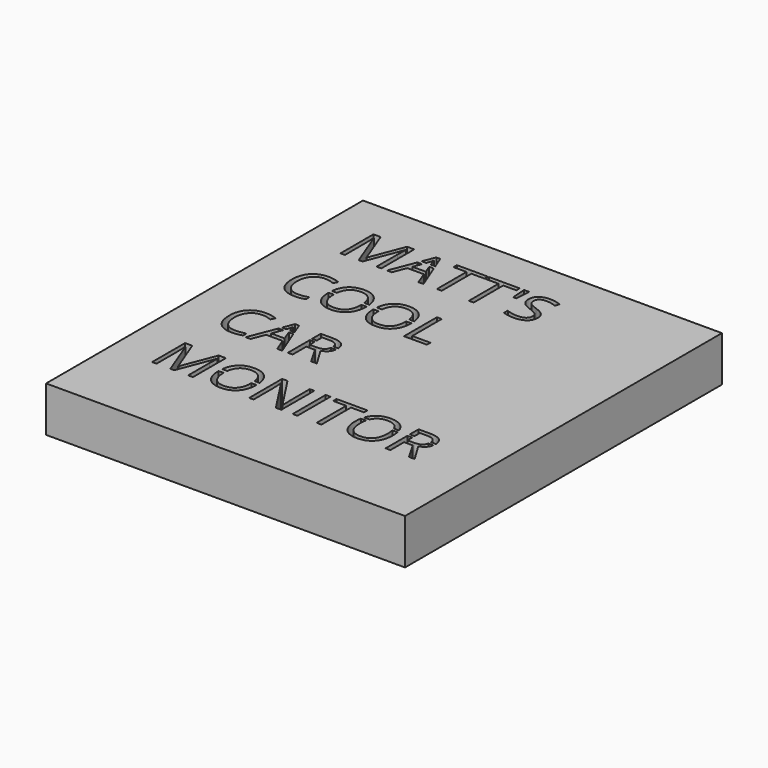
from build123d import *

# Parameters (mm, degrees)
F0_W         = 100.584
F0_H         = 110.998
F1_DEPTH     = 12.7
F2_W         = 111.76
F2_H         = 131.529821515
F2_W_2       = 100.584
F2_H_2       = 110.998
F3_DEPTH     = 10.16
F4_TEXT_SIZE = 16.1708336097
F5_DEPTH     = 25.4
F6_W         = 9.7379134968
F6_H         = 1.0117329657
F6_W_2       = 25.6726779044
F6_H_2       = 1.0865476183
F6_W_3       = 20.4207308177
F6_H_3       = 0.7884654333
F6_W_4       = 14.2759480716
F6_H_4       = 1.1968401627
F6_W_5       = 25.6291786209
F6_H_5       = 0.8507613093
F7_DEPTH     = 2.54


# Not quite as in the source:
# - a feature names something its author has since deleted; it is built from what else it names
# - Text() gives the source's letters only with a copy of the font that has no kerning and outlines rounded to 1/6400 em; it was checked with that copy


with BuildPart() as f1:
    # F0 (on Top) → F1 (new body)
    with BuildSketch(Plane.XY):
        with Locations((0, 4.191)):
            Rectangle(F0_W, F0_H)
    extrude(amount=F1_DEPTH)

    # F2 (on face) → F3 (cut)
    with BuildSketch(Plane(origin=(0, 0, 0), x_dir=(1, 0, 0), z_dir=(0, 0, -1))):
        with Locations((0, -0.4511848092)):
            Rectangle(F2_W, F2_H)
        with Locations((0, -4.191)):
            Rectangle(F2_W_2, F2_H_2, mode=Mode.SUBTRACT)
    extrude(amount=-F3_DEPTH, mode=Mode.SUBTRACT)

    # F4 (on face) → F5 (cut)
    with BuildSketch(Plane.XY.offset(12.7)):
        with Locations((-40.0829129997, 37.0636804624)):
            Text("MATT'S", F4_TEXT_SIZE, font='Open Sans', text_align=(TextAlign.LEFT, TextAlign.BOTTOM))
        with Locations((-40.0829129997, 15.0713467533)):
            Text('COOL', F4_TEXT_SIZE, font='Open Sans', text_align=(TextAlign.LEFT, TextAlign.BOTTOM))
        with Locations((-40.0829129997, -6.9209869559)):
            Text('CAR', F4_TEXT_SIZE, font='Open Sans', text_align=(TextAlign.LEFT, TextAlign.BOTTOM))
        with Locations((-40.0829129997, -28.913320665)):
            Text('MONITOR', F4_TEXT_SIZE, font='Open Sans', text_align=(TextAlign.LEFT, TextAlign.BOTTOM))
    extrude(amount=-F5_DEPTH, mode=Mode.SUBTRACT)

    # F6 (on face) → F7 (join)
    with BuildSketch(Plane.XY.offset(12.7)):
        with Locations((-19.8069675826, 44.725658372)):
            Rectangle(F6_W, F6_H)
        with Locations((-17.2776393592, 21.4184338127)):
            Rectangle(F6_W_2, F6_H_2)
        with Locations((-17.2921443811, 1.1873821204)):
            Rectangle(F6_W_3, F6_H_3)
        with Locations((-18.4418565958, -22.5426709928)):
            Rectangle(F6_W_4, F6_H_4)
        with Locations((25.4126633517, -20.8807988092)):
            Rectangle(F6_W_5, F6_H_5)
    extrude(amount=-F7_DEPTH)


solid = f1.part
